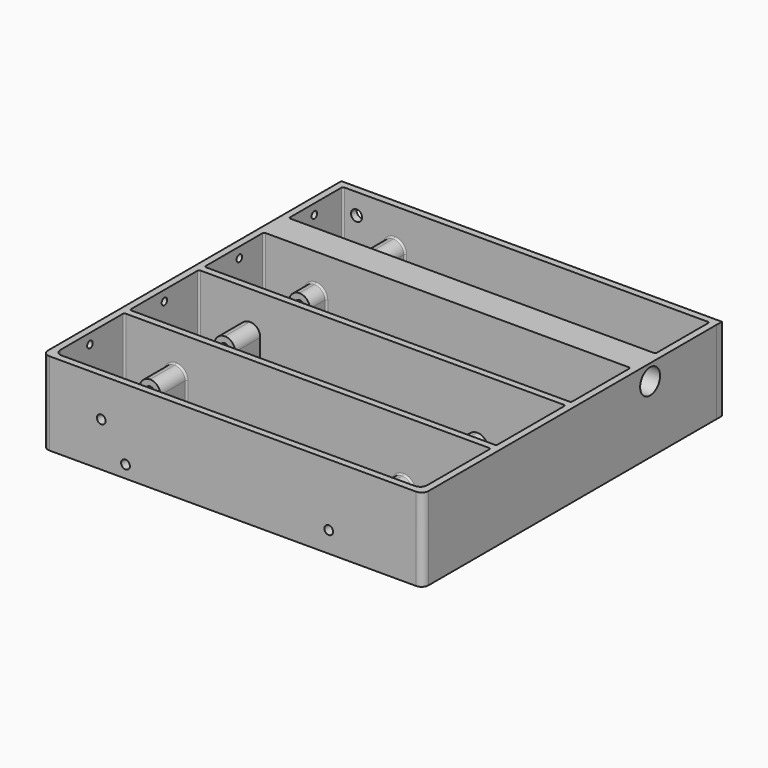
from build123d import *

# Parameters (mm, degrees)
F0_W      = 174.625
F0_H      = 174.625
F1_DEPTH  = 38.1
F2_W      = 168.275
F2_H      = 168.275
F3_DEPTH  = 34.925
F4_R      = 3.175
F5_W      = 167.9709115997
F5_H      = 3.175
F5_W_2    = 168.275
F6_DEPTH  = 38.1
F8_DEPTH  = 5.08
F10_W     = 9.525
F10_H     = 14.859
F11_DEPTH = 25.0952
F12_R     = 4.76249
F13_W     = 9.525
F13_H     = 15.5448
F14_DEPTH = 14.2875
F15_R     = 4.76249
F17_W     = 174.6388971806
F17_H     = 3.175
F18_DEPTH = 38.1
F19_W     = 174.9389618635
F19_H     = 3.8088003874
F20_DEPTH = 38.1
F21_W     = 171.2976
F21_H     = 14.2875
F22_DEPTH = 38.1
F23_R     = 0.762
F24_R     = 5.715
F25_DEPTH = 177.8
F27_W     = 5.08
F27_H     = 5.08
F28_DEPTH = 8.89
F16_R     = 2.0193
F29_DEPTH = 8.89
F26_R     = 2.0193
F30_DEPTH = 8.89
F9_R      = 1.9939
F31_DEPTH = 177.8
F32_R     = 1.5875
F33_DEPTH = 5.08
F34_R     = 2.54
F35_DEPTH = 5.08


# Not quite as in the source:
# - a fillet or chamfer is up to 0.001 mm smaller than in the source, because OpenCascade refuses the exact size


with BuildPart() as f1:
    # F0 (on Top) → F1 (new body)
    with BuildSketch(Plane.XY):
        with Locations((87.3125, 87.3125)):
            Rectangle(F0_W, F0_H)
    extrude(amount=F1_DEPTH)

    # F2 (on face) → F3 (cut)
    with BuildSketch(Plane.XY.offset(38.1)):
        with Locations((87.3125, 87.3125)):
            Rectangle(F2_W, F2_H)
    extrude(amount=-F3_DEPTH, mode=Mode.SUBTRACT)

    # F4
    f4_edges = [f1.edges().sort_by_distance(p)[0] for p in [
        (171.45, 171.45, 20.6375),
        (171.45, 3.175, 20.6375),
        (3.175, 171.45, 20.6375),
        (3.175, 3.175, 20.6375),
        (174.625, 174.625, 19.05),
        (0, 174.625, 19.05),
        (174.625, 0, 19.05),
        (0, 0, 19.05),
    ]]
    fillet(f4_edges, radius=F4_R)

    # F5 (on Top) → F6 (join)
    with BuildSketch(Plane.XY):
        with Locations((87.3412261717, 130.175)):
            Rectangle(F5_W, F5_H)
        with Locations((87.3125, 87.3125)):
            Rectangle(F5_W_2, F5_H)
        with Locations((87.3125, 44.45)):
            Rectangle(F5_W_2, F5_H)
    extrude(amount=F6_DEPTH)

    # F7 (on Top) → F8 (cut)
    with BuildSketch(Plane.XY):
        with BuildLine():
            Line((155.575, 155.0289), (73.025, 155.0289))
            ThreePointArc((73.025, 155.0289), (69.596, 151.5999), (73.025, 148.1709))
            Line((73.025, 148.1709), (155.575, 148.1709))
            ThreePointArc((155.575, 148.1709), (159.004, 151.5999), (155.575, 155.0289))
        make_face()
        with BuildLine():
            Line((73.025, 105.3211), (155.575, 105.3211))
            ThreePointArc((155.575, 105.3211), (159.004, 108.7501), (155.575, 112.1791))
            Line((155.575, 112.1791), (73.025, 112.1791))
            ThreePointArc((73.025, 112.1791), (69.596, 108.7501), (73.025, 105.3211))
        make_face()
        with BuildLine():
            Line((73.025, 62.4713), (155.575, 62.4713))
            ThreePointArc((155.575, 62.4713), (159.004, 65.9003), (155.575, 69.3293))
            Line((155.575, 69.3293), (73.025, 69.3293))
            ThreePointArc((73.025, 69.3293), (69.596, 65.9003), (73.025, 62.4713))
        make_face()
        with BuildLine():
            Line((73.025, 19.6215), (155.575, 19.6215))
            ThreePointArc((155.575, 19.6215), (159.004, 23.0505), (155.575, 26.4795))
            Line((155.575, 26.4795), (73.025, 26.4795))
            ThreePointArc((73.025, 26.4795), (69.596, 23.0505), (73.025, 19.6215))
        make_face()
    extrude(amount=F8_DEPTH, mode=Mode.SUBTRACT)

    # F10 (on Top) → F11 (join)
    with BuildSketch(Plane.XY):
        with Locations((26.9875, 10.6045)):
            Rectangle(F10_W, F10_H)
        with Locations((26.9875, 35.433)):
            Rectangle(F10_W, F10_H)
        with Locations((26.9875, 53.4543)):
            Rectangle(F10_W, F10_H)
        with Locations((26.9875, 78.2828)):
            Rectangle(F10_W, F10_H)
        with Locations((26.9875, 96.3041)):
            Rectangle(F10_W, F10_H)
        with Locations((26.9875, 121.1326)):
            Rectangle(F10_W, F10_H)
        with Locations((26.9875, 139.1539)):
            Rectangle(F10_W, F10_H)
        with Locations((26.9875, 163.9824)):
            Rectangle(F10_W, F10_H)
    extrude(amount=F11_DEPTH)

    # F12 (radius 4.7625 in the source; OpenCascade refuses exactly that, so slightly less here)
    f12_edges = [f1.edges().sort_by_distance(p)[0] for p in [
        (22.225, 163.9824, 25.0952),
        (31.75, 163.9824, 25.0952),
        (31.75, 139.17295, 25.0952),
        (22.225, 139.17295, 25.0952),
        (31.75, 121.1326, 25.0952),
        (31.75, 96.3168, 25.0952),
        (31.75, 78.2828, 25.0952),
        (31.75, 53.46065, 25.0952),
        (31.75, 35.433, 25.0952),
        (31.75, 10.6045, 25.0952),
        (22.225, 121.1326, 25.0952),
        (22.225, 78.2828, 25.0952),
        (22.225, 96.3168, 25.0952),
        (22.225, 53.46065, 25.0952),
        (22.225, 35.433, 25.0952),
        (22.225, 10.6045, 25.0952),
    ]]
    fillet(f12_edges, radius=F12_R)

    # F13 (on face) → F14 (join)
    with BuildSketch(Plane(origin=(0, 0, 0), x_dir=(1, 0, 0), z_dir=(0, 0, -1))):
        with Locations((131.3561, -10.9474)):
            Rectangle(F13_W, F13_H)
        with Locations((131.3561, -35.0901)):
            Rectangle(F13_W, F13_H)
        with Locations((131.3561, -53.7972)):
            Rectangle(F13_W, F13_H)
        with Locations((131.3561, -77.9399)):
            Rectangle(F13_W, F13_H)
        with Locations((131.3561, -96.647)):
            Rectangle(F13_W, F13_H)
        with Locations((131.3561, -120.7897)):
            Rectangle(F13_W, F13_H)
        with Locations((131.3561, -139.4968)):
            Rectangle(F13_W, F13_H)
        with Locations((131.3561, -163.6395)):
            Rectangle(F13_W, F13_H)
    extrude(amount=-F14_DEPTH)

    # F15 (radius 4.7625 in the source; OpenCascade refuses exactly that, so slightly less here)
    f15_edges = [f1.edges().sort_by_distance(p)[0] for p in [
        (126.5936, 163.6395, 14.2875),
        (126.5936, 139.51585, 14.2875),
        (126.5936, 120.7897, 14.2875),
        (126.5936, 96.6597, 14.2875),
        (126.5936, 77.9399, 14.2875),
        (126.5936, 53.80355, 14.2875),
        (126.5936, 35.0901, 14.2875),
        (126.5936, 10.9474, 14.2875),
        (136.1186, 10.9474, 14.2875),
        (136.1186, 35.0901, 14.2875),
        (136.1186, 53.80355, 14.2875),
        (136.1186, 77.9399, 14.2875),
        (136.1186, 96.6597, 14.2875),
        (136.1186, 120.7897, 14.2875),
        (136.1186, 139.51585, 14.2875),
        (136.1186, 163.6395, 14.2875),
    ]]
    fillet(f15_edges, radius=F15_R)

    # F17 (on Top) → F18 (join)
    with BuildSketch(Plane.XY):
        with Locations((87.3194485903, 169.8625)):
            Rectangle(F17_W, F17_H)
    extrude(amount=F18_DEPTH)

    # F19 (on Top) → F20 (cut)
    with BuildSketch(Plane.XY):
        with Locations((87.4694809318, 173.3544001937)):
            Rectangle(F19_W, F19_H)
    extrude(amount=F20_DEPTH, mode=Mode.SUBTRACT)

    # F21 (on Top) → F22 (join)
    with BuildSketch(Plane.XY):
        with Locations((88.2789392626, 130.16865)):
            Rectangle(F21_W, F21_H)
    extrude(amount=F22_DEPTH)

    # F23
    f23_edges = [f1.edges().sort_by_distance(p)[0] for p in [
        (31.75, 168.275, 11.753855),
        (136.1186, 168.275, 6.350005),
        (127.988501, 168.275, 12.892599),
        (126.5936, 168.275, 6.350005),
        (31.75, 137.3124, 11.753855),
        (126.5936, 137.3124, 6.350005),
        (31.75, 123.0249, 11.753855),
        (136.1186, 123.0249, 6.350005),
        (136.1186, 85.7123, 6.350005),
        (31.75, 85.7123, 11.753855),
        (31.75, 42.8625, 11.753855),
        (136.1186, 42.8625, 6.350005),
        (3.175, 42.8625, 20.6375),
        (3.175, 85.725, 20.6375),
        (3.175, 123.0249, 20.6375),
        (171.45, 168.275, 20.6375),
        (171.45, 123.0249, 20.6375),
        (171.45, 85.725, 20.6375),
        (171.45, 42.8625, 20.6375),
        (136.1186, 88.9, 6.350005),
        (31.75, 88.9, 11.753855),
        (31.75, 46.0375, 11.753855),
        (136.1186, 46.0375, 6.350005),
        (136.1186, 3.175, 6.350005),
        (31.75, 3.175, 11.753855),
        (3.175, 46.0375, 20.6375),
        (3.175, 88.9, 20.6375),
        (171.45, 46.0375, 20.6375),
        (171.45, 88.9, 20.6375),
        (171.45, 137.3124, 20.6375),
        (3.175, 168.275, 20.6375),
        (3.175, 137.3124, 20.6375),
    ]]
    fillet(f23_edges, radius=F23_R)

    # F24 (on face) → F25 (cut)
    with BuildSketch(Plane(origin=(0, 0, 0), x_dir=(0, -1, 0), z_dir=(-1, 0, 0))):
        with Locations((-130.2791535854, 30.7504776865)):
            Circle(F24_R)
    extrude(amount=-F25_DEPTH, mode=Mode.SUBTRACT)

    # F27 (on face) → F28 (join)
    with BuildSketch(Plane(origin=(0, 0, 0), x_dir=(1, 0, 0), z_dir=(0, 0, -1))):
        with Locations((38.1, -5.715)):
            Rectangle(F27_W, F27_H)
        with Locations((38.1, -165.735)):
            Rectangle(F27_W, F27_H)
    extrude(amount=-F28_DEPTH)

    # F16 (on face) → F29 (cut)
    with BuildSketch(Plane.XZ):
        with Locations((38.1, 5.715)):
            Circle(F16_R)
    extrude(amount=-F29_DEPTH, mode=Mode.SUBTRACT)

    # F26 (on face) → F30 (cut)
    with BuildSketch(Plane(origin=(0, 171.45, 0), x_dir=(-1, 0, 0), z_dir=(0, 1, 0))):
        with Locations((-38.0533486605, 5.715)):
            Circle(F26_R)
    extrude(amount=-F30_DEPTH, mode=Mode.SUBTRACT)

    # F9 (on face) → F31 (cut)
    with BuildSketch(Plane.XZ):
        with Locations((131.3561, 9.525)):
            Circle(F9_R)
        with Locations((26.9875, 20.32)):
            Circle(F9_R)
    extrude(amount=-F31_DEPTH, mode=Mode.SUBTRACT)

    # F32 (on face) → F33 (cut)
    with BuildSketch(Plane(origin=(0, 0, 0), x_dir=(0, -1, 0), z_dir=(-1, 0, 0))):
        with Locations((-151.985630393, 33.3804748952)):
            Circle(F32_R)
        with Locations((-108.972735703, 33.3804748952)):
            Circle(F32_R)
        with Locations((-65.959841013, 33.3804748952)):
            Circle(F32_R)
        with Locations((-23.2477318496, 33.3804748952)):
            Circle(F32_R)
    extrude(amount=-F33_DEPTH, mode=Mode.SUBTRACT)

    # F34 (on face) → F35 (cut)
    with BuildSketch(Plane(origin=(0, 171.45, 0), x_dir=(-1, 0, 0), z_dir=(0, 1, 0))):
        with Locations((-9.525, 28.575)):
            Circle(F34_R)
        with Locations((-165.1138971806, 28.575)):
            Circle(F34_R)
    extrude(amount=-F35_DEPTH, mode=Mode.SUBTRACT)


solid = f1.part
